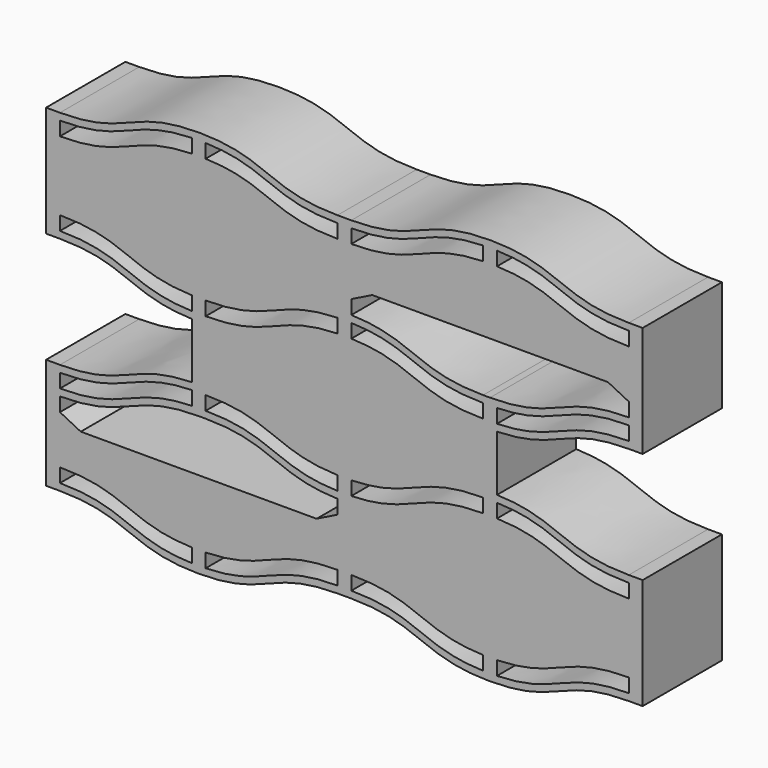
from build123d import *

# Parameters (mm, degrees)
F1_DEPTH = 25


with BuildPart() as f1:
    # F0 (on Front) → F1 (new body)
    with BuildSketch(Plane.XZ):
        with BuildLine():
            add(Edge.make_bspline(
                [(110.25, -4e-10), (101.5, -4e-10), (93.051839448, 3.3792642203), (84.6036788961, 6.7585284411), (77, 6.9755853243)],
                knots=[0, 0, 0, 0, 0.5, 0.9655040631, 0.9655040631, 0.9655040631, 0.9655040631], degree=3))
            Line((77, 6.9755853243), (77, 21.0244146753))
            add(Edge.make_bspline(
                [(77, 21.0244146753), (84.6036788961, 21.2414715584), (93.051839448, 24.6207357792), (101.5, 28), (110.25, 28)],
                knots=[0.0344959369, 0.0344959369, 0.0344959369, 0.0344959369, 0.5, 1, 1, 1, 1], degree=3))
            Line((110.25, 28), (113.75, 28))
            Line((113.75, 28), (113.75, 55.9999999996))
            Line((113.75, 55.9999999996), (110.25, 55.9999999996))
            add(Edge.make_bspline(
                [(110.25, 56), (101.5, 56), (92.75, 59.5), (84, 63), (75.25, 63)],
                knots=[0, 0, 0, 0, 0.5, 1, 1, 1, 1], degree=3))
            add(Edge.make_bspline(
                [(75.25, 63), (66.5, 63), (57.75, 59.5), (49, 56), (40.25, 56)],
                knots=[0, 0, 0, 0, 0.5, 1, 1, 1, 1], degree=3))
            Line((40.25, 56), (36.75, 56))
            add(Edge.make_bspline(
                [(36.75, 56.0000000004), (28, 56.0000000004), (19.25, 59.5000000004), (10.5, 63.0000000004), (1.75, 63.0000000004)],
                knots=[0, 0, 0, 0, 0.5, 1, 1, 1, 1], degree=3))
            add(Edge.make_bspline(
                [(1.75, 63.0000000004), (-7, 63.0000000004), (-15.75, 59.5000000004), (-24.5, 56.0000000004), (-33.25, 56.0000000004)],
                knots=[0, 0, 0, 0, 0.5, 1, 1, 1, 1], degree=3))
            Line((-33.25, 56.0000000004), (-36.75, 56.0000000004))
            Line((-36.75, 56.0000000004), (-36.75, 28.0000000004))
            Line((-36.75, 28.0000000004), (-33.25, 28.0000000004))
            add(Edge.make_bspline(
                [(-33.25, 28.0000000004), (-24.5, 28.0000000004), (-16.051839448, 24.6207357797), (-7.6036788961, 21.2414715589), (0, 21.0244146757)],
                knots=[0, 0, 0, 0, 0.5, 0.9655040631, 0.9655040631, 0.9655040631, 0.9655040631], degree=3))
            Line((0, 21.0244146757), (0, 6.9755853247))
            add(Edge.make_bspline(
                [(0, 6.9755853247), (-7.6036788961, 6.7585284416), (-16.051839448, 3.3792642208), (-24.5, 0), (-33.25, 0)],
                knots=[0.0344959369, 0.0344959369, 0.0344959369, 0.0344959369, 0.5, 1, 1, 1, 1], degree=3))
            Line((-33.25, 0), (-36.75, 0))
            Line((-36.75, 0), (-36.75, -27.9999999996))
            Line((-36.75, -27.9999999996), (-33.25, -27.9999999996))
            add(Edge.make_bspline(
                [(-33.25, -28), (-24.5, -28), (-15.75, -31.5), (-7, -35), (1.75, -35)],
                knots=[0, 0, 0, 0, 0.5, 1, 1, 1, 1], degree=3))
            add(Edge.make_bspline(
                [(1.75, -35), (10.5, -35), (19.25, -31.5), (28, -28), (36.75, -28)],
                knots=[0, 0, 0, 0, 0.5, 1, 1, 1, 1], degree=3))
            Line((36.75, -28), (40.25, -28))
            add(Edge.make_bspline(
                [(40.25, -28.0000000004), (49, -28.0000000004), (57.75, -31.5000000004), (66.5, -35.0000000004), (75.25, -35.0000000004)],
                knots=[0, 0, 0, 0, 0.5, 1, 1, 1, 1], degree=3))
            add(Edge.make_bspline(
                [(75.25, -35.0000000004), (84, -35.0000000004), (92.75, -31.5000000004), (101.5, -28.0000000004), (110.25, -28.0000000004)],
                knots=[0, 0, 0, 0, 0.5, 1, 1, 1, 1], degree=3))
            Line((110.25, -28.0000000004), (113.75, -28.0000000004))
            Line((113.75, -28.0000000004), (113.75, -4e-10))
            Line((113.75, -4e-10), (110.25, -4e-10))
        make_face()
        with BuildLine():
            add(Edge.make_bspline(
                [(-33.25, -26.25), (-24.5, -26.25), (-16.051839448, -29.6292642208), (-7.6036788961, -33.0085284416), (0, -33.2255853247)],
                knots=[0, 0, 0, 0, 0.5, 0.9655040631, 0.9655040631, 0.9655040631, 0.9655040631], degree=3))
            Line((-33.25, -26.2499999996), (-33.25, -22.7499999996))
            add(Edge.make_bspline(
                [(-33.25, -22.75), (-24.5, -22.75), (-16.051839448, -26.1292642208), (-7.6036788961, -29.5085284416), (0, -29.7255853247)],
                knots=[0, 0, 0, 0, 0.5, 0.9655040631, 0.9655040631, 0.9655040631, 0.9655040631], degree=3))
            add(Edge.make_bspline(
                [(0, -29.7255853247), (0.563466677, -29.7416702124), (1.1463211039, -29.75), (1.75, -29.75)],
                knots=[0.9655040631, 0.9655040631, 0.9655040631, 0.9655040631, 1, 1, 1, 1], degree=3))
            add(Edge.make_bspline(
                [(1.75, -29.75), (2.3536788961, -29.75), (2.936533323, -29.7416702124), (3.5, -29.7255853247)],
                knots=[0, 0, 0, 0, 0.0344959369, 0.0344959369, 0.0344959369, 0.0344959369], degree=3))
            add(Edge.make_bspline(
                [(3.5, -29.7255853247), (11.1036788961, -29.5085284416), (19.551839448, -26.1292642208), (28, -22.75), (36.75, -22.75)],
                knots=[0.0344959369, 0.0344959369, 0.0344959369, 0.0344959369, 0.5, 1, 1, 1, 1], degree=3))
            Line((36.75, -22.75), (36.75, -26.25))
            add(Edge.make_bspline(
                [(3.5, -33.2255853247), (11.1036788961, -33.0085284416), (19.551839448, -29.6292642208), (28, -26.25), (36.75, -26.25)],
                knots=[0.0344959369, 0.0344959369, 0.0344959369, 0.0344959369, 0.5, 1, 1, 1, 1], degree=3))
            add(Edge.make_bspline(
                [(1.75, -33.25), (2.3536788961, -33.25), (2.936533323, -33.2416702124), (3.5, -33.2255853247)],
                knots=[0, 0, 0, 0, 0.0344959369, 0.0344959369, 0.0344959369, 0.0344959369], degree=3))
            add(Edge.make_bspline(
                [(0, -33.2255853247), (0.563466677, -33.2416702124), (1.1463211039, -33.25), (1.75, -33.25)],
                knots=[0.9655040631, 0.9655040631, 0.9655040631, 0.9655040631, 1, 1, 1, 1], degree=3))
        make_face(mode=Mode.SUBTRACT)
        with BuildLine():
            add(Edge.make_bspline(
                [(-33.25, -5.25), (-24.5, -5.25), (-16.051839448, -1.8707357792), (-7.6036788961, 1.5085284416), (0, 1.7255853247)],
                knots=[0, 0, 0, 0, 0.5, 0.9655040631, 0.9655040631, 0.9655040631, 0.9655040631], degree=3))
            Line((-33.25, -5.2499999996), (-33.25, -1.7499999996))
            add(Edge.make_bspline(
                [(-33.25, -1.75), (-24.5, -1.75), (-16.051839448, 1.6292642208), (-7.6036788961, 5.0085284416), (0, 5.2255853247)],
                knots=[0, 0, 0, 0, 0.5, 0.9655040631, 0.9655040631, 0.9655040631, 0.9655040631], degree=3))
            Line((0, 5.2255853247), (0, 3.5267737359))
            Line((0, 3.5267737359), (0, 1.7255853247))
        make_face(mode=Mode.SUBTRACT)
        with BuildLine():
            Line((1.75, 0), (3.5, 0))
            add(Edge.make_bspline(
                [(3.5, 0), (12.25, 0), (20.698160552, -3.3792642208), (29.1463211039, -6.7585284416), (36.75, -6.9755853247)],
                knots=[0, 0, 0, 0, 0.5, 0.9655040631, 0.9655040631, 0.9655040631, 0.9655040631], degree=3))
            Line((36.75, -6.9755853247), (36.75, -7))
            Line((36.75, -7), (36.75, -10.5))
            Line((36.75, -10.5), (31.5, -13.125))
            Line((31.5, -13.125), (-28, -13.125))
            Line((-28, -13.125), (-33.25, -10.5))
            Line((-33.25, -10.4999999996), (-33.25, -6.9999999996))
            add(Edge.make_bspline(
                [(-33.25, -7), (-24.5, -7), (-15.75, -3.5), (-7, 0), (1.75, 0)],
                knots=[0, 0, 0, 0, 0.5, 1, 1, 1, 1], degree=3))
        make_face(mode=Mode.SUBTRACT)
        with BuildLine():
            add(Edge.make_bspline(
                [(40.25, -26.2500000004), (49, -26.2500000004), (57.448160552, -29.6292642212), (65.8963211039, -33.008528442), (73.5, -33.2255853252)],
                knots=[0, 0, 0, 0, 0.5, 0.9655040631, 0.9655040631, 0.9655040631, 0.9655040631], degree=3))
            Line((40.25, -26.25), (40.25, -22.75))
            add(Edge.make_bspline(
                [(40.25, -22.7500000004), (49, -22.7500000004), (57.448160552, -26.1292642212), (65.8963211039, -29.508528442), (73.5, -29.7255853252)],
                knots=[0, 0, 0, 0, 0.5, 0.9655040631, 0.9655040631, 0.9655040631, 0.9655040631], degree=3))
            add(Edge.make_bspline(
                [(73.5, -29.7255853252), (74.063466677, -29.7416702128), (74.6463211039, -29.7500000004), (75.25, -29.7500000004)],
                knots=[0.9655040631, 0.9655040631, 0.9655040631, 0.9655040631, 1, 1, 1, 1], degree=3))
            add(Edge.make_bspline(
                [(75.25, -29.7500000004), (75.8536788961, -29.7500000004), (76.436533323, -29.7416702128), (77, -29.7255853252)],
                knots=[0, 0, 0, 0, 0.0344959369, 0.0344959369, 0.0344959369, 0.0344959369], degree=3))
            add(Edge.make_bspline(
                [(77, -29.7255853252), (84.6036788961, -29.508528442), (93.051839448, -26.1292642212), (101.5, -22.7500000004), (110.25, -22.7500000004)],
                knots=[0.0344959369, 0.0344959369, 0.0344959369, 0.0344959369, 0.5, 1, 1, 1, 1], degree=3))
            Line((110.25, -22.7500000004), (110.25, -26.2500000004))
            add(Edge.make_bspline(
                [(77, -33.2255853252), (84.6036788961, -33.008528442), (93.051839448, -29.6292642212), (101.5, -26.2500000004), (110.25, -26.2500000004)],
                knots=[0.0344959369, 0.0344959369, 0.0344959369, 0.0344959369, 0.5, 1, 1, 1, 1], degree=3))
            add(Edge.make_bspline(
                [(75.25, -33.2500000004), (75.8536788961, -33.2500000004), (76.436533323, -33.2416702128), (77, -33.2255853252)],
                knots=[0, 0, 0, 0, 0.0344959369, 0.0344959369, 0.0344959369, 0.0344959369], degree=3))
            add(Edge.make_bspline(
                [(73.5, -33.2255853252), (74.063466677, -33.2416702128), (74.6463211039, -33.2500000004), (75.25, -33.2500000004)],
                knots=[0.9655040631, 0.9655040631, 0.9655040631, 0.9655040631, 1, 1, 1, 1], degree=3))
        make_face(mode=Mode.SUBTRACT)
        with BuildLine():
            add(Edge.make_bspline(
                [(73.5, 5.25), (64.75, 5.25), (56.301839448, 1.8707357792), (47.8536788961, -1.5085284416), (40.25, -1.7255853247)],
                knots=[0, 0, 0, 0, 0.5, 0.9655040631, 0.9655040631, 0.9655040631, 0.9655040631], degree=3))
            Line((73.5, 5.2499999996), (73.5, 5.2255853243))
            Line((73.5, 5.2255853243), (73.5, 3.5267737355))
            Line((73.5, 3.5267737355), (73.5, 1.7499999996))
            add(Edge.make_bspline(
                [(73.5, 1.75), (64.75, 1.75), (56.301839448, -1.6292642208), (47.8536788961, -5.0085284416), (40.25, -5.2255853247)],
                knots=[0, 0, 0, 0, 0.5, 0.9655040631, 0.9655040631, 0.9655040631, 0.9655040631], degree=3))
            add(Edge.make_bspline(
                [(40.25, -5.2255853247), (39.686533323, -5.2416702124), (39.1036788961, -5.25), (38.5, -5.25)],
                knots=[0.9655040631, 0.9655040631, 0.9655040631, 0.9655040631, 1, 1, 1, 1], degree=3))
            add(Edge.make_bspline(
                [(36.75, -5.2255853247), (37.313466677, -5.2416702124), (37.8963211039, -5.25), (38.5, -5.25)],
                knots=[0.9655040631, 0.9655040631, 0.9655040631, 0.9655040631, 1, 1, 1, 1], degree=3))
            add(Edge.make_bspline(
                [(3.5, 1.75), (12.25, 1.75), (20.698160552, -1.6292642208), (29.1463211039, -5.0085284416), (36.75, -5.2255853247)],
                knots=[0, 0, 0, 0, 0.5, 0.9655040631, 0.9655040631, 0.9655040631, 0.9655040631], degree=3))
            Line((3.5, 1.75), (3.5, 3.5267737359))
            Line((3.5, 3.5267737359), (3.5, 5.2255853247))
            Line((3.5, 5.2255853247), (3.5, 5.25))
            add(Edge.make_bspline(
                [(36.75, -1.7255853247), (29.1463211039, -1.5085284416), (20.698160552, 1.8707357792), (12.25, 5.25), (3.5, 5.25)],
                knots=[0.0344959369, 0.0344959369, 0.0344959369, 0.0344959369, 0.5, 1, 1, 1, 1], degree=3))
            add(Edge.make_bspline(
                [(38.5, -1.75), (37.8963211039, -1.75), (37.313466677, -1.7416702124), (36.75, -1.7255853247)],
                knots=[0, 0, 0, 0, 0.0344959369, 0.0344959369, 0.0344959369, 0.0344959369], degree=3))
            add(Edge.make_bspline(
                [(40.25, -1.7255853247), (39.686533323, -1.7416702124), (39.1036788961, -1.75), (38.5, -1.75)],
                knots=[0.9655040631, 0.9655040631, 0.9655040631, 0.9655040631, 1, 1, 1, 1], degree=3))
        make_face(mode=Mode.SUBTRACT)
        with BuildLine():
            add(Edge.make_bspline(
                [(77, 1.7255853243), (84.6036788961, 1.5085284411), (93.051839448, -1.8707357797), (101.5, -5.2500000004), (110.25, -5.2500000004)],
                knots=[0.0344959369, 0.0344959369, 0.0344959369, 0.0344959369, 0.5, 1, 1, 1, 1], degree=3))
            Line((77, 1.7255853243), (77, 3.5267737355))
            Line((77, 3.5267737355), (77, 5.2255853243))
            add(Edge.make_bspline(
                [(110.25, -1.7500000004), (101.5, -1.7500000004), (93.051839448, 1.6292642203), (84.6036788961, 5.0085284411), (77, 5.2255853243)],
                knots=[0, 0, 0, 0, 0.5, 0.9655040631, 0.9655040631, 0.9655040631, 0.9655040631], degree=3))
            Line((110.25, -1.7500000004), (110.25, -5.2500000004))
        make_face(mode=Mode.SUBTRACT)
        with BuildLine():
            add(Edge.make_bspline(
                [(0, 26.2744146757), (-7.6036788961, 26.4914715589), (-16.051839448, 29.8707357797), (-24.5, 33.2500000004), (-33.25, 33.2500000004)],
                knots=[0.0344959369, 0.0344959369, 0.0344959369, 0.0344959369, 0.5, 1, 1, 1, 1], degree=3))
            Line((0, 26.2744146757), (0, 24.4732262646))
            Line((0, 24.4732262646), (0, 22.7744146757))
            add(Edge.make_bspline(
                [(-33.25, 29.7500000004), (-24.5, 29.7500000004), (-16.051839448, 26.3707357797), (-7.6036788961, 22.9914715589), (0, 22.7744146757)],
                knots=[0, 0, 0, 0, 0.5, 0.9655040631, 0.9655040631, 0.9655040631, 0.9655040631], degree=3))
            Line((-33.25, 29.7500000004), (-33.25, 33.2500000004))
        make_face(mode=Mode.SUBTRACT)
        with BuildLine():
            add(Edge.make_bspline(
                [(36.75, 54.2500000004), (28, 54.2500000004), (19.551839448, 57.6292642212), (11.1036788961, 61.008528442), (3.5, 61.2255853252)],
                knots=[0, 0, 0, 0, 0.5, 0.9655040631, 0.9655040631, 0.9655040631, 0.9655040631], degree=3))
            Line((36.75, 54.25), (36.75, 50.75))
            add(Edge.make_bspline(
                [(36.75, 50.7500000004), (28, 50.7500000004), (19.551839448, 54.1292642212), (11.1036788961, 57.508528442), (3.5, 57.7255853252)],
                knots=[0, 0, 0, 0, 0.5, 0.9655040631, 0.9655040631, 0.9655040631, 0.9655040631], degree=3))
            add(Edge.make_bspline(
                [(3.5, 57.7255853252), (2.936533323, 57.7416702128), (2.3536788961, 57.7500000004), (1.75, 57.7500000004)],
                knots=[0.9655040631, 0.9655040631, 0.9655040631, 0.9655040631, 1, 1, 1, 1], degree=3))
            add(Edge.make_bspline(
                [(1.75, 57.7500000004), (1.1463211039, 57.7500000004), (0.563466677, 57.7416702128), (0, 57.7255853252)],
                knots=[0, 0, 0, 0, 0.0344959369, 0.0344959369, 0.0344959369, 0.0344959369], degree=3))
            add(Edge.make_bspline(
                [(0, 57.7255853252), (-7.6036788961, 57.508528442), (-16.051839448, 54.1292642212), (-24.5, 50.7500000004), (-33.25, 50.7500000004)],
                knots=[0.0344959369, 0.0344959369, 0.0344959369, 0.0344959369, 0.5, 1, 1, 1, 1], degree=3))
            Line((-33.25, 50.7500000004), (-33.25, 54.2500000004))
            add(Edge.make_bspline(
                [(0, 61.2255853252), (-7.6036788961, 61.008528442), (-16.051839448, 57.6292642212), (-24.5, 54.2500000004), (-33.25, 54.2500000004)],
                knots=[0.0344959369, 0.0344959369, 0.0344959369, 0.0344959369, 0.5, 1, 1, 1, 1], degree=3))
            add(Edge.make_bspline(
                [(1.75, 61.2500000004), (1.1463211039, 61.2500000004), (0.563466677, 61.2416702128), (0, 61.2255853252)],
                knots=[0, 0, 0, 0, 0.0344959369, 0.0344959369, 0.0344959369, 0.0344959369], degree=3))
            add(Edge.make_bspline(
                [(3.5, 61.2255853252), (2.936533323, 61.2416702128), (2.3536788961, 61.2500000004), (1.75, 61.2500000004)],
                knots=[0.9655040631, 0.9655040631, 0.9655040631, 0.9655040631, 1, 1, 1, 1], degree=3))
        make_face(mode=Mode.SUBTRACT)
        with BuildLine():
            add(Edge.make_bspline(
                [(73.5, 26.25), (64.75, 26.25), (56.301839448, 29.6292642208), (47.8536788961, 33.0085284416), (40.25, 33.2255853247)],
                knots=[0, 0, 0, 0, 0.5, 0.9655040631, 0.9655040631, 0.9655040631, 0.9655040631], degree=3))
            Line((73.5, 26.2499999996), (73.5, 24.4732262641))
            Line((73.5, 24.4732262641), (73.5, 22.7744146753))
            Line((73.5, 22.7744146753), (73.5, 22.7499999996))
            add(Edge.make_bspline(
                [(73.5, 22.75), (64.75, 22.75), (56.301839448, 26.1292642208), (47.8536788961, 29.5085284416), (40.25, 29.7255853247)],
                knots=[0, 0, 0, 0, 0.5, 0.9655040631, 0.9655040631, 0.9655040631, 0.9655040631], degree=3))
            add(Edge.make_bspline(
                [(40.25, 29.7255853247), (39.686533323, 29.7416702124), (39.1036788961, 29.75), (38.5, 29.75)],
                knots=[0.9655040631, 0.9655040631, 0.9655040631, 0.9655040631, 1, 1, 1, 1], degree=3))
            add(Edge.make_bspline(
                [(38.5, 29.75), (37.8963211039, 29.75), (37.313466677, 29.7416702124), (36.75, 29.7255853247)],
                knots=[0, 0, 0, 0, 0.0344959369, 0.0344959369, 0.0344959369, 0.0344959369], degree=3))
            add(Edge.make_bspline(
                [(36.75, 29.7255853247), (29.1463211039, 29.5085284416), (20.698160552, 26.1292642208), (12.25, 22.75), (3.5, 22.75)],
                knots=[0.0344959369, 0.0344959369, 0.0344959369, 0.0344959369, 0.5, 1, 1, 1, 1], degree=3))
            Line((3.5, 22.75), (3.5, 22.7744146757))
            Line((3.5, 22.7744146757), (3.5, 24.4732262645))
            Line((3.5, 24.4732262645), (3.5, 26.25))
            add(Edge.make_bspline(
                [(36.75, 33.2255853247), (29.1463211039, 33.0085284416), (20.698160552, 29.6292642208), (12.25, 26.25), (3.5, 26.25)],
                knots=[0.0344959369, 0.0344959369, 0.0344959369, 0.0344959369, 0.5, 1, 1, 1, 1], degree=3))
            add(Edge.make_bspline(
                [(38.5, 33.25), (37.8963211039, 33.25), (37.313466677, 33.2416702124), (36.75, 33.2255853247)],
                knots=[0, 0, 0, 0, 0.0344959369, 0.0344959369, 0.0344959369, 0.0344959369], degree=3))
            add(Edge.make_bspline(
                [(40.25, 33.2255853247), (39.686533323, 33.2416702124), (39.1036788961, 33.25), (38.5, 33.25)],
                knots=[0.9655040631, 0.9655040631, 0.9655040631, 0.9655040631, 1, 1, 1, 1], degree=3))
        make_face(mode=Mode.SUBTRACT)
        with BuildLine():
            Line((75.25, 28), (73.5, 28))
            add(Edge.make_bspline(
                [(73.5, 28), (64.75, 28), (56.301839448, 31.3792642208), (47.8536788961, 34.7585284416), (40.25, 34.9755853247)],
                knots=[0, 0, 0, 0, 0.5, 0.9655040631, 0.9655040631, 0.9655040631, 0.9655040631], degree=3))
            Line((40.25, 34.9755853247), (40.25, 35))
            Line((40.25, 35), (40.25, 38.5))
            Line((40.25, 38.5), (45.5, 41.125))
            Line((45.5, 41.125), (105, 41.125))
            Line((105, 41.125), (110.25, 38.5))
            Line((110.25, 38.4999999996), (110.25, 34.9999999996))
            add(Edge.make_bspline(
                [(110.25, 35), (101.5, 35), (92.75, 31.5), (84, 28), (75.25, 28)],
                knots=[0, 0, 0, 0, 0.5, 1, 1, 1, 1], degree=3))
        make_face(mode=Mode.SUBTRACT)
        with BuildLine():
            add(Edge.make_bspline(
                [(110.25, 33.25), (101.5, 33.25), (93.051839448, 29.8707357792), (84.6036788961, 26.4914715584), (77, 26.2744146753)],
                knots=[0, 0, 0, 0, 0.5, 0.9655040631, 0.9655040631, 0.9655040631, 0.9655040631], degree=3))
            Line((110.25, 33.2499999996), (110.25, 29.7499999996))
            add(Edge.make_bspline(
                [(110.25, 29.75), (101.5, 29.75), (93.051839448, 26.3707357792), (84.6036788961, 22.9914715584), (77, 22.7744146753)],
                knots=[0, 0, 0, 0, 0.5, 0.9655040631, 0.9655040631, 0.9655040631, 0.9655040631], degree=3))
            Line((77, 22.7744146753), (77, 24.4732262641))
            Line((77, 24.4732262641), (77, 26.2744146753))
        make_face(mode=Mode.SUBTRACT)
        with BuildLine():
            add(Edge.make_bspline(
                [(110.25, 54.25), (101.5, 54.25), (93.051839448, 57.6292642208), (84.6036788961, 61.0085284416), (77, 61.2255853247)],
                knots=[0, 0, 0, 0, 0.5, 0.9655040631, 0.9655040631, 0.9655040631, 0.9655040631], degree=3))
            Line((110.25, 54.2499999996), (110.25, 50.7499999996))
            add(Edge.make_bspline(
                [(110.25, 50.75), (101.5, 50.75), (93.051839448, 54.1292642208), (84.6036788961, 57.5085284416), (77, 57.7255853247)],
                knots=[0, 0, 0, 0, 0.5, 0.9655040631, 0.9655040631, 0.9655040631, 0.9655040631], degree=3))
            add(Edge.make_bspline(
                [(77, 57.7255853247), (76.436533323, 57.7416702124), (75.8536788961, 57.75), (75.25, 57.75)],
                knots=[0.9655040631, 0.9655040631, 0.9655040631, 0.9655040631, 1, 1, 1, 1], degree=3))
            add(Edge.make_bspline(
                [(75.25, 57.75), (74.6463211039, 57.75), (74.063466677, 57.7416702124), (73.5, 57.7255853247)],
                knots=[0, 0, 0, 0, 0.0344959369, 0.0344959369, 0.0344959369, 0.0344959369], degree=3))
            add(Edge.make_bspline(
                [(73.5, 57.7255853247), (65.8963211039, 57.5085284416), (57.448160552, 54.1292642208), (49, 50.75), (40.25, 50.75)],
                knots=[0.0344959369, 0.0344959369, 0.0344959369, 0.0344959369, 0.5, 1, 1, 1, 1], degree=3))
            Line((40.25, 50.75), (40.25, 54.25))
            add(Edge.make_bspline(
                [(73.5, 61.2255853247), (65.8963211039, 61.0085284416), (57.448160552, 57.6292642208), (49, 54.25), (40.25, 54.25)],
                knots=[0.0344959369, 0.0344959369, 0.0344959369, 0.0344959369, 0.5, 1, 1, 1, 1], degree=3))
            add(Edge.make_bspline(
                [(75.25, 61.25), (74.6463211039, 61.25), (74.063466677, 61.2416702124), (73.5, 61.2255853247)],
                knots=[0, 0, 0, 0, 0.0344959369, 0.0344959369, 0.0344959369, 0.0344959369], degree=3))
            add(Edge.make_bspline(
                [(77, 61.2255853247), (76.436533323, 61.2416702124), (75.8536788961, 61.25), (75.25, 61.25)],
                knots=[0.9655040631, 0.9655040631, 0.9655040631, 0.9655040631, 1, 1, 1, 1], degree=3))
        make_face(mode=Mode.SUBTRACT)
        with BuildLine():
            Line((40.25, -1.7500000002), (40.25, -1.7255853247))
            add(Edge.make_bspline(
                [(40.25, -1.7255853247), (39.686533323, -1.7416702124), (39.1036788961, -1.75), (38.5, -1.75)],
                knots=[0.9655040631, 0.9655040631, 0.9655040631, 0.9655040631, 1, 1, 1, 1], degree=3))
            add(Edge.make_bspline(
                [(38.5, -1.75), (37.8963211039, -1.75), (37.313466677, -1.7416702124), (36.75, -1.7255853247)],
                knots=[0, 0, 0, 0, 0.0344959369, 0.0344959369, 0.0344959369, 0.0344959369], degree=3))
            Line((36.75, -1.7255853247), (36.75, -1.75))
            Line((36.75, -1.75), (36.75, -3.5267737359))
            Line((36.75, -3.5267737359), (36.75, -5.2255853247))
            add(Edge.make_bspline(
                [(36.75, -5.2255853247), (37.313466677, -5.2416702124), (37.8963211039, -5.25), (38.5, -5.25)],
                knots=[0.9655040631, 0.9655040631, 0.9655040631, 0.9655040631, 1, 1, 1, 1], degree=3))
            add(Edge.make_bspline(
                [(40.25, -5.2255853247), (39.686533323, -5.2416702124), (39.1036788961, -5.25), (38.5, -5.25)],
                knots=[0.9655040631, 0.9655040631, 0.9655040631, 0.9655040631, 1, 1, 1, 1], degree=3))
            Line((40.25, -5.2255853247), (40.25, -3.5267737359))
            Line((40.25, -3.5267737359), (40.25, -1.7500000002))
        make_face()
        with BuildLine():
            Line((40.25, 31.5267588347), (40.25, 33.2255853247))
            add(Edge.make_bspline(
                [(40.25, 33.2255853247), (39.686533323, 33.2416702124), (39.1036788961, 33.25), (38.5, 33.25)],
                knots=[0.9655040631, 0.9655040631, 0.9655040631, 0.9655040631, 1, 1, 1, 1], degree=3))
            add(Edge.make_bspline(
                [(38.5, 33.25), (37.8963211039, 33.25), (37.313466677, 33.2416702124), (36.75, 33.2255853247)],
                knots=[0, 0, 0, 0, 0.0344959369, 0.0344959369, 0.0344959369, 0.0344959369], degree=3))
            Line((36.75, 33.2255853247), (36.75, 29.7500000002))
            Line((36.75, 29.7500000002), (36.75, 29.7255853247))
            add(Edge.make_bspline(
                [(38.5, 29.75), (37.8963211039, 29.75), (37.313466677, 29.7416702124), (36.75, 29.7255853247)],
                knots=[0, 0, 0, 0, 0.0344959369, 0.0344959369, 0.0344959369, 0.0344959369], degree=3))
            add(Edge.make_bspline(
                [(40.25, 29.7255853247), (39.686533323, 29.7416702124), (39.1036788961, 29.75), (38.5, 29.75)],
                knots=[0.9655040631, 0.9655040631, 0.9655040631, 0.9655040631, 1, 1, 1, 1], degree=3))
            Line((40.25, 29.7255853247), (40.25, 29.75))
            Line((40.25, 29.75), (40.25, 31.5267588347))
        make_face()
        with BuildLine():
            Line((77, 59.5267588347), (77, 61.2255853247))
            add(Edge.make_bspline(
                [(77, 61.2255853247), (76.436533323, 61.2416702124), (75.8536788961, 61.25), (75.25, 61.25)],
                knots=[0.9655040631, 0.9655040631, 0.9655040631, 0.9655040631, 1, 1, 1, 1], degree=3))
            add(Edge.make_bspline(
                [(75.25, 61.25), (74.6463211039, 61.25), (74.063466677, 61.2416702124), (73.5, 61.2255853247)],
                knots=[0, 0, 0, 0, 0.0344959369, 0.0344959369, 0.0344959369, 0.0344959369], degree=3))
            Line((73.5, 61.2255853247), (73.5, 57.7255853247))
            add(Edge.make_bspline(
                [(75.25, 57.75), (74.6463211039, 57.75), (74.063466677, 57.7416702124), (73.5, 57.7255853247)],
                knots=[0, 0, 0, 0, 0.0344959369, 0.0344959369, 0.0344959369, 0.0344959369], degree=3))
            add(Edge.make_bspline(
                [(77, 57.7255853247), (76.436533323, 57.7416702124), (75.8536788961, 57.75), (75.25, 57.75)],
                knots=[0.9655040631, 0.9655040631, 0.9655040631, 0.9655040631, 1, 1, 1, 1], degree=3))
            Line((77, 57.7255853247), (77, 59.5267588347))
        make_face()
        with BuildLine():
            Line((3.5, 59.5267588352), (3.5, 61.2255853252))
            add(Edge.make_bspline(
                [(3.5, 61.2255853252), (2.936533323, 61.2416702128), (2.3536788961, 61.2500000004), (1.75, 61.2500000004)],
                knots=[0.9655040631, 0.9655040631, 0.9655040631, 0.9655040631, 1, 1, 1, 1], degree=3))
            add(Edge.make_bspline(
                [(1.75, 61.2500000004), (1.1463211039, 61.2500000004), (0.563466677, 61.2416702128), (0, 61.2255853252)],
                knots=[0, 0, 0, 0, 0.0344959369, 0.0344959369, 0.0344959369, 0.0344959369], degree=3))
            Line((0, 61.2255853252), (0, 57.7255853252))
            add(Edge.make_bspline(
                [(1.75, 57.7500000004), (1.1463211039, 57.7500000004), (0.563466677, 57.7416702128), (0, 57.7255853252)],
                knots=[0, 0, 0, 0, 0.0344959369, 0.0344959369, 0.0344959369, 0.0344959369], degree=3))
            add(Edge.make_bspline(
                [(3.5, 57.7255853252), (2.936533323, 57.7416702128), (2.3536788961, 57.7500000004), (1.75, 57.7500000004)],
                knots=[0.9655040631, 0.9655040631, 0.9655040631, 0.9655040631, 1, 1, 1, 1], degree=3))
            Line((3.5, 57.7255853252), (3.5, 59.5267588352))
        make_face()
        with BuildLine():
            Line((0, -31.5267588347), (0, -33.2255853247))
            add(Edge.make_bspline(
                [(0, -33.2255853247), (0.563466677, -33.2416702124), (1.1463211039, -33.25), (1.75, -33.25)],
                knots=[0.9655040631, 0.9655040631, 0.9655040631, 0.9655040631, 1, 1, 1, 1], degree=3))
            add(Edge.make_bspline(
                [(1.75, -33.25), (2.3536788961, -33.25), (2.936533323, -33.2416702124), (3.5, -33.2255853247)],
                knots=[0, 0, 0, 0, 0.0344959369, 0.0344959369, 0.0344959369, 0.0344959369], degree=3))
            Line((3.5, -33.2255853247), (3.5, -29.7255853247))
            add(Edge.make_bspline(
                [(1.75, -29.75), (2.3536788961, -29.75), (2.936533323, -29.7416702124), (3.5, -29.7255853247)],
                knots=[0, 0, 0, 0, 0.0344959369, 0.0344959369, 0.0344959369, 0.0344959369], degree=3))
            add(Edge.make_bspline(
                [(0, -29.7255853247), (0.563466677, -29.7416702124), (1.1463211039, -29.75), (1.75, -29.75)],
                knots=[0.9655040631, 0.9655040631, 0.9655040631, 0.9655040631, 1, 1, 1, 1], degree=3))
            Line((0, -29.7255853247), (0, -31.5267588347))
        make_face()
        with BuildLine():
            Line((73.5, -31.5267588352), (73.5, -33.2255853252))
            add(Edge.make_bspline(
                [(73.5, -33.2255853252), (74.063466677, -33.2416702128), (74.6463211039, -33.2500000004), (75.25, -33.2500000004)],
                knots=[0.9655040631, 0.9655040631, 0.9655040631, 0.9655040631, 1, 1, 1, 1], degree=3))
            add(Edge.make_bspline(
                [(75.25, -33.2500000004), (75.8536788961, -33.2500000004), (76.436533323, -33.2416702128), (77, -33.2255853252)],
                knots=[0, 0, 0, 0, 0.0344959369, 0.0344959369, 0.0344959369, 0.0344959369], degree=3))
            Line((77, -33.2255853252), (77, -29.7255853252))
            add(Edge.make_bspline(
                [(75.25, -29.7500000004), (75.8536788961, -29.7500000004), (76.436533323, -29.7416702128), (77, -29.7255853252)],
                knots=[0, 0, 0, 0, 0.0344959369, 0.0344959369, 0.0344959369, 0.0344959369], degree=3))
            add(Edge.make_bspline(
                [(73.5, -29.7255853252), (74.063466677, -29.7416702128), (74.6463211039, -29.7500000004), (75.25, -29.7500000004)],
                knots=[0.9655040631, 0.9655040631, 0.9655040631, 0.9655040631, 1, 1, 1, 1], degree=3))
            Line((73.5, -29.7255853252), (73.5, -31.5267588352))
        make_face()
    extrude(amount=F1_DEPTH)


solid = f1.part
